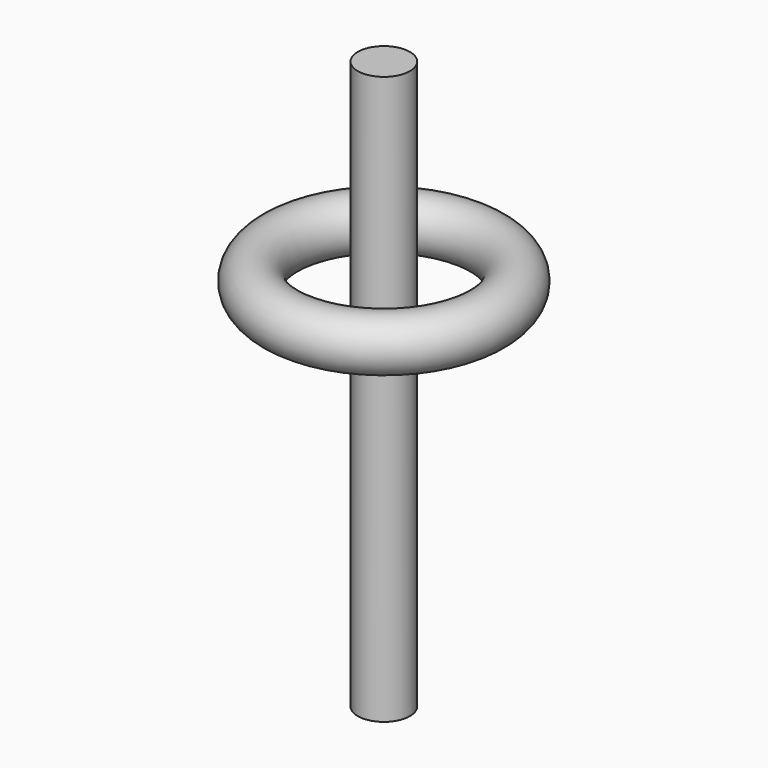
from build123d import *

# Parameters (mm, degrees)
F0_R          = 9.3293252752
F3_R          = 9.3293243603
F4_DEPTH      = 101.6
F4_DEPTH_BACK = 101.6


# Not quite as in the source:
# - the program builds the solid bodies; features that only make, move or delete a surface that nothing else refers to are left out


with BuildPart() as f2:
    # F0 (on Front) → F2 (revolve)
    with BuildSketch(Plane.XZ):
        with Locations((-36.9971059263, 32.4852652848)):
            Circle(F0_R)
    revolve(axis=Axis((0, 0, 12.4827632681), (0, 0, -1)))


with BuildPart() as f4:
    # F3 (on Top) → F4 (new body, two sides)
    with BuildSketch(Plane.XY) as f4_sk:
        Circle(F3_R)
    extrude(amount=F4_DEPTH)
    extrude(f4_sk.sketch, amount=-F4_DEPTH_BACK)


solid = Compound([f2.part, f4.part])
